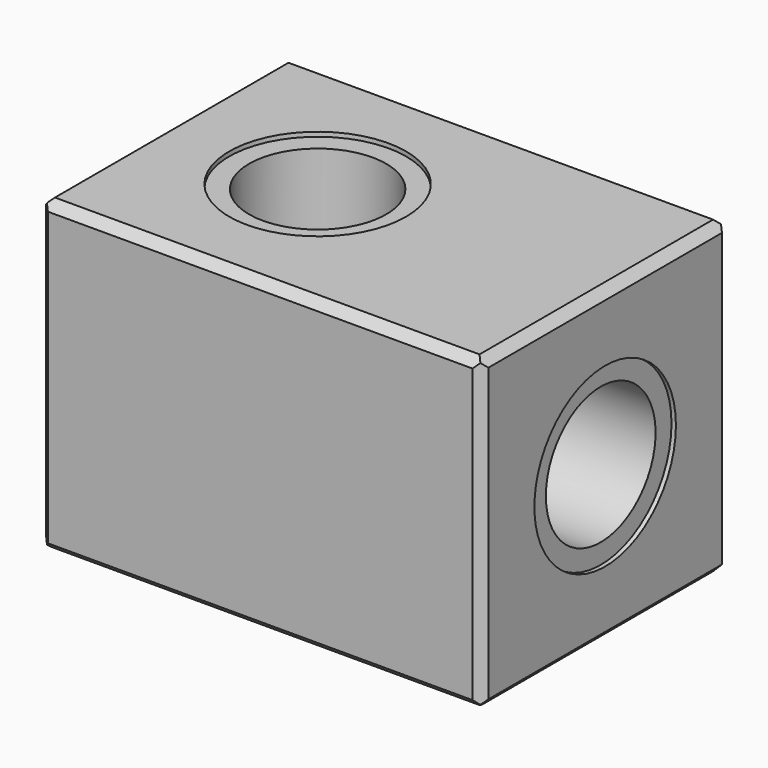
from build123d import *

# Parameters (mm, degrees)
F0_W         = 50
F0_H         = 35
F1_DEPTH     = 35
F3_D         = 15.5
F3_DEPTH     = 18
F3_TIP       = 4.6566697975
F5_D         = 15.5
F5_DEPTH     = 18
F5_TIP       = 4.6566697975
F7_D         = 8
F7_DEPTH     = 33
F7_TIP       = 2.4034424761
F8_R         = 10
F8_R_2       = 7.75
F9_DEPTH     = 0.5
F10_R        = 10
F10_R_2      = 7.75
F11_DEPTH    = 0.5
F13_SIZE     = 1
F14_T1_DEPTH = 39.1433659759
F14_T3_DEPTH = 39.1433659759
F14_T5_DEPTH = 55.1433659759
F14_T7_DEPTH = 50.2571417204


# Not quite as in the source:
# - a fillet or chamfer that OpenCascade refuses, or shapes differently, is made with other operations: its cross-section is extruded or revolved along the edge and cut away or added
# - a feature of the source that left no trace in its solid (it failed there, or was rolled back) is left out


with BuildPart() as f1:
    # F0 (on Front) → F1 (new body)
    with BuildSketch(Plane.XZ):
        with Locations((25, 17.5)):
            Rectangle(F0_W, F0_H)
    extrude(amount=F1_DEPTH)

    # F3
    with Locations(Plane.YZ.offset(50)):
        with Locations((-17.5, 17.5)):
            Hole(F3_D / 2, depth=F3_DEPTH)
            with Locations((0, 0, -(F3_DEPTH + F3_TIP / 2))):  # 118° drill point
                Cone(0, F3_D / 2, F3_TIP, mode=Mode.SUBTRACT)

    # F5
    with Locations(Plane.XY.offset(35)):
        with Locations((17.5, -17.5)):
            Hole(F5_D / 2, depth=F5_DEPTH)
            with Locations((0, 0, -(F5_DEPTH + F5_TIP / 2))):  # 118° drill point
                Cone(0, F5_D / 2, F5_TIP, mode=Mode.SUBTRACT)

    # F7
    with Locations(Plane.YZ.offset(50)):
        with Locations((-17.5, 17.5)):
            Hole(F7_D / 2, depth=F7_DEPTH)
            with Locations((0, 0, -(F7_DEPTH + F7_TIP / 2))):  # 118° drill point
                Cone(0, F7_D / 2, F7_TIP, mode=Mode.SUBTRACT)

    # F8 (on face) → F9 (cut)
    with BuildSketch(Plane.YZ.offset(50)):
        with Locations((-17.5, 17.5)):
            Circle(F8_R)
        with Locations((-17.5, 17.5)):
            Circle(F8_R_2, mode=Mode.SUBTRACT)
    extrude(amount=-F9_DEPTH, mode=Mode.SUBTRACT)

    # F10 (on face) → F11 (cut)
    with BuildSketch(Plane.XY.offset(35)):
        with Locations((17.5, -17.5)):
            Circle(F10_R)
        with Locations((17.5, -17.5)):
            Circle(F10_R_2, mode=Mode.SUBTRACT)
    extrude(amount=-F11_DEPTH, mode=Mode.SUBTRACT)

    # F13
    f13_edges = [f1.edges().sort_by_distance(p)[0] for p in [
        (0, 0, 17.5),
        (25, 0, 0),
        (50, 0, 17.5),
        (25, 0, 35),
        (0, -17.5, 0),
        (50, -17.5, 0),
        (25, -35, 0),
    ]]
    chamfer(f13_edges, length=F13_SIZE)

    # F14: chamfer of 1 on 6 edges, made by hand

    # F14_s2 → F14_t1 (cut)
    with BuildSketch(Plane.XZ.offset(-1.571682988)):
        Polygon((0, 34), (1, 35), (0, 35), align=None)
        Polygon((49, 35), (50, 34), (50, 35), align=None)
    extrude(amount=F14_T1_DEPTH, mode=Mode.SUBTRACT)

    # F14_s4 → F14_t3 (cut)
    with BuildSketch(Plane.XY.offset(-1.571682988)):
        Polygon((0, -34), (1, -35), (0, -35), align=None)
        Polygon((49, -35), (50, -34), (50, -35), align=None)
    extrude(amount=F14_T3_DEPTH, mode=Mode.SUBTRACT)

    # F14_s6 → F14_t5 (cut)
    with BuildSketch(Plane.YZ.offset(-2.571682988)):
        Polygon((-34, 35), (-35, 34), (-35, 35), align=None)
    extrude(amount=F14_T5_DEPTH, mode=Mode.SUBTRACT)

    # F14_s8 → F14_t7 (cut)
    with BuildSketch(Plane.YZ.offset(-0.1285708602)):
        Polygon((-34.2928932188, 0.2928932188), (-33.5857864376, 0), (-34, 0), align=None)
    extrude(amount=F14_T7_DEPTH, mode=Mode.SUBTRACT)


solid = f1.part
